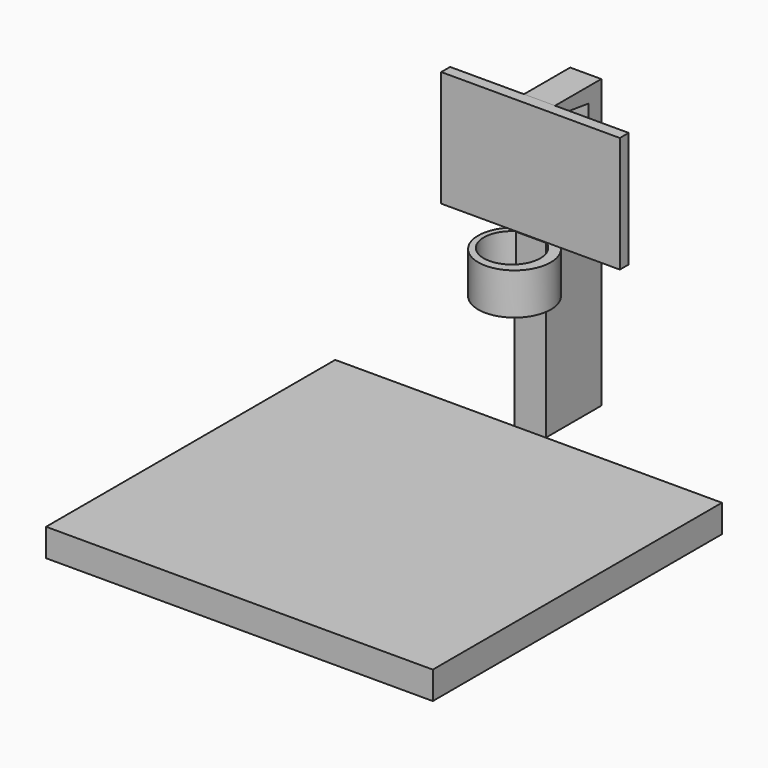
from build123d import *

# Parameters (mm, degrees)
F0_W      = 139.5270854934
F0_H      = 130.3940266371
F1_DEPTH  = 10
F3_DEPTH  = 4
F4_W      = 11.2278764136
F4_H      = 61.8974082172
F5_DEPTH  = 25
F6_W      = 11.2278764136
F6_H      = 41.8618817022
F7_DEPTH  = 22
F9_DEPTH  = 25
F11_DEPTH = 15
F13_DEPTH = 25


with BuildPart() as f1:
    # F0 (on Top) → F1 (new body)
    with BuildSketch(Plane.XY):
        with Locations((-0.2840146073, 0.2853274345)):
            Rectangle(F0_W, F0_H)
    extrude(amount=-F1_DEPTH)


with BuildPart() as f3:
    # F2 (on face) → F3 (new body)
    with BuildSketch(Plane(origin=(0, 65.4823407531, 0), x_dir=(-1, 0, 0), z_dir=(0, 1, 0))):
        Polygon((-32.6489694417, 62.0584264398), (-6.1345105059, 62.0584264398), (5.2785333246, 62.0584264398), (31.7929922603, 62.0584264398), (31.7929922603, 103.8682609797), (-32.6489694417, 103.8682609797), align=None)
    extrude(amount=F3_DEPTH)



with BuildPart() as f5:
    # F4 (on face) → F5 (new body)
    with BuildSketch(Plane(origin=(0, 65.4823407531, 0), x_dir=(-1, 0, 0), z_dir=(0, 1, 0))):
        with Locations((-0.3402393777, 30.9487041086)):
            Rectangle(F4_W, F4_H)
    extrude(amount=F5_DEPTH)


with BuildPart() as f7:
    # F6 (on face) → F7 (new body)
    with BuildSketch(Plane(origin=(0, 90.4823407531, 0), x_dir=(-1, 0, 0), z_dir=(0, 1, 0))):
        with Locations((-0.3402393777, 82.8283490683)):
            Rectangle(F6_W, F6_H)
    extrude(amount=-F7_DEPTH)

    # F8 (on face) → F9 (cut)
    with BuildSketch(Plane.YZ.offset(5.9541775845)):
        Polygon((84.8051980138, 61.8974082172), (84.8051980138, 98.3029305935), (69.4944635034, 100.4393099771), (69.4944635034, 61.8974082172), align=None)
    extrude(amount=-F9_DEPTH, mode=Mode.SUBTRACT)


with BuildPart() as f3_1:
    add(f3.part)

    add(f5.part)  # F11 merges F5
    # F10 (on face) → F11 (join)
    with BuildSketch(Plane(origin=(0, 0, 62.0584264398), x_dir=(1, 0, 0), z_dir=(0, 0, -1))):
        with BuildLine():
            Line((-8.2063768059, -65.4823407531), (11.3937389106, -65.4823407531))
            ThreePointArc((11.3937389106, -65.4823407531), (1.5936810523, -43.7000604931), (-8.2063768059, -65.4823407531))
        make_face()
    extrude(amount=F11_DEPTH)

    # F12 (on face) → F13 (cut)
    with BuildSketch(Plane.XY.offset(62.0584264398)):
        with BuildLine():
            Line((6.1381380074, 65.4823407531), (-4.8790327273, 65.4823407531))
            ThreePointArc((-4.8790327273, 65.4823407531), (0.62955264, 46.6897500929), (6.1381380074, 65.4823407531))
        make_face()
    extrude(amount=-F13_DEPTH, mode=Mode.SUBTRACT)


solid = Compound([f1.part, f7.part, f3_1.part])
